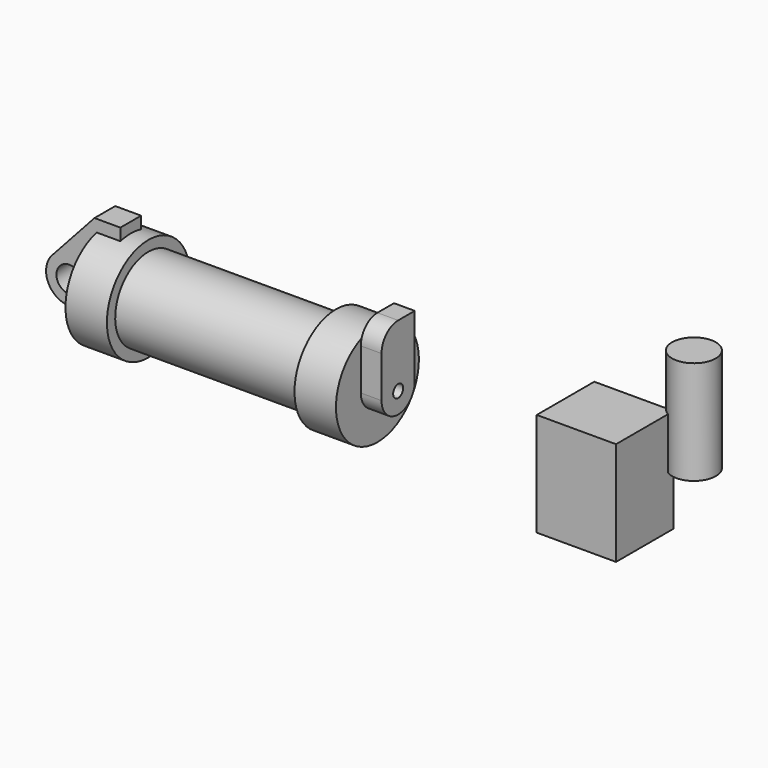
from build123d import *

# Parameters (mm, degrees)
F0_W        = 0.23
F0_H        = 0.5
F0_R        = 0.125
F2_DEPTH    = 0.125
F3_R        = 0.06
F4_DEPTH    = 0.2
F5_T1_DEPTH = 0.7
F6_W        = 0.7649799809
F6_H        = 0.6938194565
F7_DEPTH    = 0.5
F8_R        = 0.2112818978
F9_DEPTH    = 1


# Not quite as in the source:
# - a fillet or chamfer that OpenCascade refuses, or shapes differently, is made with other operations: its cross-section is extruded or revolved along the edge and cut away or added


with BuildPart() as f1:
    # F0 (on Front) → F1 (revolve)
    with BuildSketch(Plane.XZ):
        with Locations((0.115, 0.25)):
            Rectangle(F0_W, F0_H)
        Polygon((0.4, 0.5), (0.23, 0.5), (0.23, 0), (2.61, 0), (2.61, 0.5), (2.21, 0.5), (2.21, 0.4), (0.4, 0.4), align=None)
    revolve(axis=Axis((1.305, 0, 0), (1, 0, 0)))

    # F0 (on Front) → F2 (join, symmetric)
    with BuildSketch(Plane.XZ):
        with Locations((0.115, 0.25)):
            Rectangle(F0_W, F0_H)
        with BuildLine():
            Line((0, 0), (0, 0.5))
            Line((0, 0.5), (0.23, 0.5))
            Line((0.23, 0.5), (0.23, 0.6))
            Line((0.23, 0.6), (-0.02, 0.6))
            Line((-0.02, 0.6), (-0.4283712527, 0.1514780719))
            ThreePointArc((-0.4283712527, 0.1514780719), (-0.1807858752, 0.209831518), (-0.037, 0))
            ThreePointArc((-0.037, 0), (-0.1258185404, -0.1791078169), (-0.3221520895, -0.216810346))
            Line((-0.3221520895, -0.216810346), (0.23, -0.37))
            Line((0.23, -0.37), (0.23, 0))
            Line((0.23, 0), (0, 0))
        make_face()
        with BuildLine():
            ThreePointArc((-0.037, 0), (-0.1807858752, 0.209831518), (-0.4283712527, 0.1514780719))
            ThreePointArc((-0.4283712527, 0.1514780719), (-0.4781881029, -0.0623514568), (-0.3221520895, -0.216810346))
            ThreePointArc((-0.3221520895, -0.216810346), (-0.1258185404, -0.1791078169), (-0.037, 0))
        make_face()
        with Locations((-0.262, 0)):
            Circle(F0_R, mode=Mode.SUBTRACT)
    extrude(amount=F2_DEPTH, both=True)

    # F3 (on face) → F4 (join)
    with BuildSketch(Plane.YZ.offset(2.61)):
        with BuildLine():
            ThreePointArc((-0.2, 0), (0, 0.2), (0.2, 0))
            Line((0.2, 0), (0.2, 0.4582575695))
            ThreePointArc((0.2, 0.4582575695), (0, 0.5), (-0.2, 0.4582575695))
            Line((-0.2, 0.4582575695), (-0.2, 0))
        make_face()
        with BuildLine():
            ThreePointArc((-0.2, 0.4582575695), (0, 0.5), (0.2, 0.4582575695))
            Line((0.2, 0.4582575695), (0.2, 0.6))
            Line((0.2, 0.6), (-0.2, 0.6))
            Line((-0.2, 0.6), (-0.2, 0.4582575695))
        make_face()
        with BuildLine():
            ThreePointArc((-0.2, 0), (0, -0.2), (0.2, 0))
            ThreePointArc((0.2, 0), (0, 0.2), (-0.2, 0))
        make_face()
        Circle(F3_R, mode=Mode.SUBTRACT)
    extrude(amount=F4_DEPTH)

    # F5: fillet of radius 0.2 on 1 edges, made by hand

    # F5_s2 → F5_t1 (cut)
    with BuildSketch(Plane.YZ.offset(2.61)):
        with BuildLine():
            ThreePointArc((-0.2, 0.4), (-0.1414213562, 0.5414213562), (0, 0.6))
            Line((0, 0.6), (-0.2, 0.6))
            Line((-0.2, 0.6), (-0.2, 0.4))
        make_face()
    extrude(amount=F5_T1_DEPTH, mode=Mode.SUBTRACT)


with BuildPart() as f7:
    # F6 (on Top) → F7 (new body, symmetric)
    with BuildSketch(Plane.XY):
        with Locations((4.8514064401, -0.0550320692)):
            Rectangle(F6_W, F6_H)
    extrude(amount=F7_DEPTH, both=True)


with BuildPart() as f9:
    # F8 (on Top) → F9 (new body)
    with BuildSketch(Plane.XY):
        with Locations((5.6408504024, 0.2423605474)):
            Circle(F8_R)
    extrude(amount=F9_DEPTH)


with BuildPart() as f9_1:
    # F10: moved
    add(f9.part.moved(Location((-0.30558, 0.16855, 0))))


solid = Compound([f1.part, f7.part, f9_1.part])
